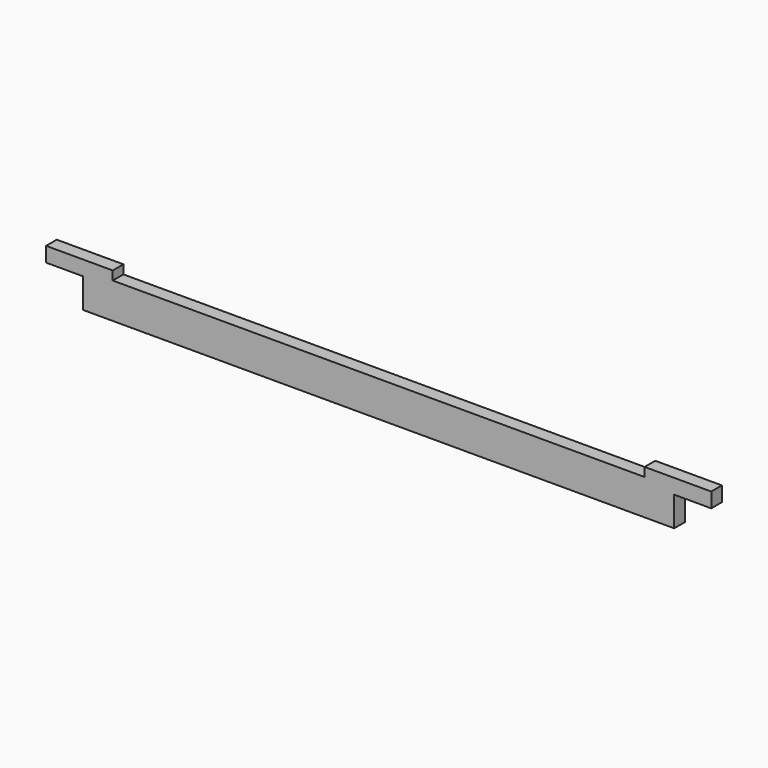
from build123d import *

# Parameters (mm, degrees)
F1_DEPTH = 18


# Not quite as in the source:
# - a feature names something its author has since deleted; it is built from what else it names


with BuildPart() as f1:
    # F0 (on Front) → F1 (new body)
    with BuildSketch(Plane.XZ):
        Polygon((0, 20), (0, 0), (50, 0), (50, -40), (848, -40), (848, 0), (898, 0), (898, 20), (808, 20), (808, 8), (90, 8), (90, 20), align=None)
    extrude(amount=F1_DEPTH)


solid = f1.part
